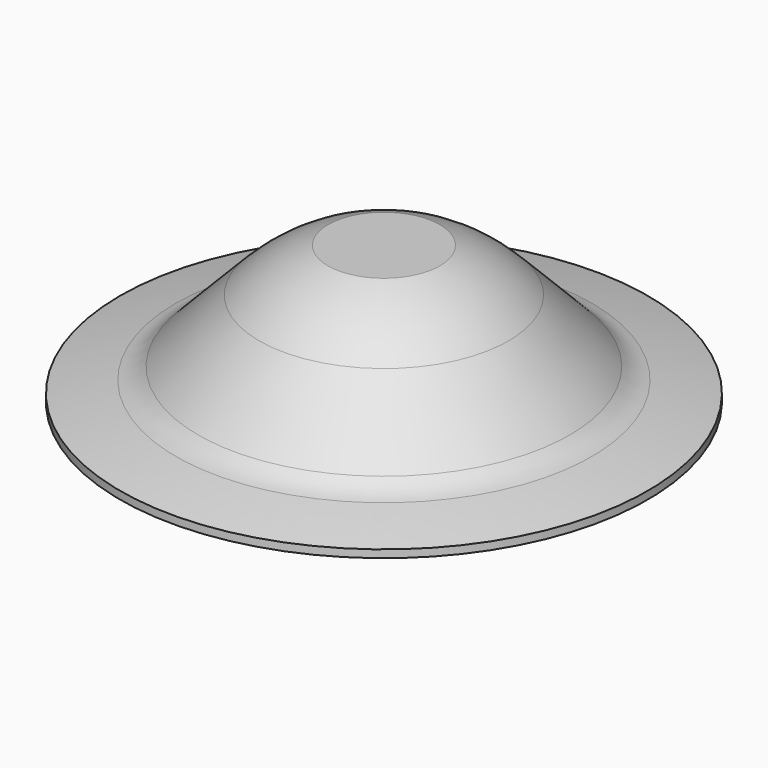
from build123d import *

# Parameters (mm, degrees)
F3_DEPTH = 12.5


with BuildPart() as f1:
    # F0 (on Front) → F1 (revolve)
    with BuildSketch(Plane.XZ):
        with BuildLine():
            ThreePointArc((-18.0916087155, 2.4896269549), (-9.0697101385, 3.4763084496), (0, 3.8057812268))
            Line((0, 3.8057812268), (0, 15.685))
            ThreePointArc((0, 15.685), (-7.408626068, 14.1810641227), (-13.6443996575, 9.9073431353))
            ThreePointArc((-13.6443996575, 9.9073431353), (-16.295679955, 6.4548932852), (-18.0916087155, 2.4896269549))
        make_face()
        with BuildLine():
            ThreePointArc((-21.3346085291, 1.9716631865), (-19.7148097422, 2.2412958765), (-18.0916087155, 2.4896269549))
            ThreePointArc((-18.0916087155, 2.4896269549), (-16.295679955, 6.4548932852), (-13.6443996575, 9.9073431353))
            Line((-13.6443996575, 9.9073431353), (-20.3248404986, 3.0136629614))
            Line((-20.3248404986, 3.0136629614), (-21.3346085291, 1.9716631865))
        make_face()
        with BuildLine():
            ThreePointArc((-22.7378459416, 1.7203465229), (-25.8145491381, 1.1111738013), (-28.875, 0.425))
            Line((-28.875, 0.425), (-18.6282688407, 0.425))
            ThreePointArc((-18.6282688407, 0.425), (-18.3889375183, 1.464851143), (-18.0916087155, 2.4896269549))
            ThreePointArc((-18.0916087155, 2.4896269549), (-19.7148097422, 2.2412958765), (-21.3346085291, 1.9716631865))
            ThreePointArc((-21.3346085291, 1.9716631865), (-22.0365855065, 1.848005277), (-22.7378459416, 1.7203465229))
        make_face()
        Polygon((-28.875, -0.425), (0, -0.425), (0, 0), (0, 0.425), (-18.6282688407, 0.425), (-28.875, 0.425), align=None)
        with BuildLine():
            ThreePointArc((-20.3248404986, 3.0136629614), (-21.4306013049, 2.1790454907), (-22.7378459416, 1.7203465229))
            ThreePointArc((-22.7378459416, 1.7203465229), (-22.0365855065, 1.848005277), (-21.3346085291, 1.9716631865))
            Line((-21.3346085291, 1.9716631865), (-20.3248404986, 3.0136629614))
        make_face()
        with BuildLine():
            Line((-18.6282688407, 0.425), (0, 0.425))
            Line((0, 0.425), (0, 3.8057812268))
            ThreePointArc((0, 3.8057812268), (-9.0697101385, 3.4763084496), (-18.0916087155, 2.4896269549))
            ThreePointArc((-18.0916087155, 2.4896269549), (-18.3889375183, 1.464851143), (-18.6282688407, 0.425))
        make_face()
    revolve(axis=Axis((0, 0, 10.397832983), (0, 0, 1)))

    # F2 (on Right) → F3 (cut, symmetric)
    with BuildSketch(Plane.YZ):
        Polygon((-34.8162702815, 14.675), (27.6827993542, 14.675), (-3.9353072157, 26.7957725373), (-36.1574023472, 14.675), align=None)
    extrude(amount=F3_DEPTH, both=True, mode=Mode.SUBTRACT)


solid = f1.part
